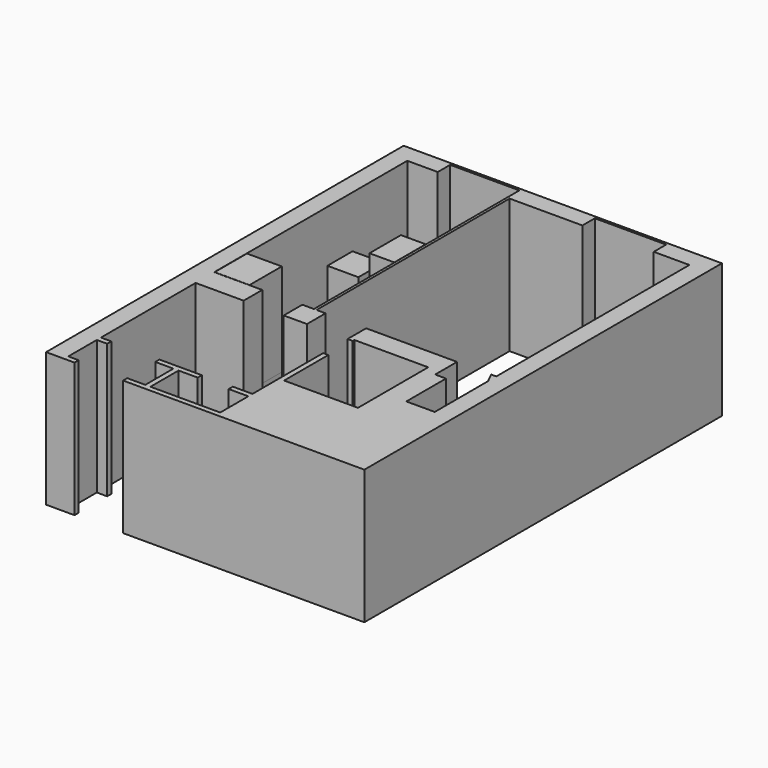
from build123d import *

# Parameters (mm, degrees)
F1_DEPTH = 800
F0_W     = 430
F0_H     = 1300
F0_W_2   = 220
F0_H_2   = 720
F0_W_3   = 480
F0_H_3   = 1200
F0_H_4   = 760
F0_W_4   = 675
F0_H_5   = 780
F0_W_5   = 600
F0_H_6   = 531.0021286011
F0_H_7   = 100
F0_H_8   = 1304.4725608826
F0_H_9   = 607.3201847076
F0_W_6   = 642.8868770599
F0_H_10  = 620.1963424683
F2_DEPTH = 1200
F3_DEPTH = 800
F4_DEPTH = 1800


with BuildPart() as f1:
    # F0 (on Top) → F1 (new body)
    with BuildSketch(Plane.XY):
        Polygon((0, -3630), (0, 5020), (-6160, 5020), (-6160, -3630), (-5810, -3630), (-5610, -3630), (-5610, -3530), (-5810, -3530), (-5810, -2840), (-5610, -2840), (-5610, -2740), (-5810, -2740), (-5810, -450), (-4880, -450), (-4880, 0), (-5810, 0), (-5810, 4670), (-5220, 4670), (-5220, 4970), (-3880, 4970), (-3880, 4670), (-3880, 0), (-4105, 0), (-4105, -450), (-3655, -450), (-3655, 0), (-3830, 0), (-3830, 4670), (-2420, 4670), (-2420, 4970), (-1040, 4970), (-1040, 4670), (-350, 4670), (-350, 0), (-450, 0), (-350, -200), (-350, -1490), (-900, -1490), (-900, -530), (-1110, -530), (-1110, 0), (-2870, 0), (-2870, -450), (-2770, -450), (-2770, -410), (-1340, -410), (-1340, -2110), (-2770, -2110), (-2770, -1040), (-2870, -1040), (-2870, -2750), (-3250, -2750), (-3250, -2850), (-2870, -2850), (-2870, -3530), (-4220, -3530), (-4220, -2850), (-3850, -2850), (-3850, -2750), (-4670, -2750), (-4670, -2850), (-4320, -2850), (-4320, -3530), (-4670, -3530), (-4670, -3630), (-4320, -3630), align=None)
    extrude(amount=F1_DEPTH)

    # F4 (add): a face of the model
    f4_faces = [f1.faces().sort_by_distance(p)[0] for p in [
        (-2581.1160504996, -299.791944949, 800),
    ]]
    extrude(f4_faces, amount=F4_DEPTH)


with BuildPart() as f1b:
    # F0 (on Top) → F1, piece 2 (new body)
    with BuildSketch(Plane.XY):
        with Locations((-3095, -1790)):
            Rectangle(F0_W, F0_H)
    extrude(amount=F1_DEPTH)

    # F2 (add): a face of the model
    f2_faces = [f1b.faces().sort_by_distance(p)[0] for p in [
        (-3095, -1790, 800),
    ]]
    extrude(f2_faces, amount=F2_DEPTH)


with BuildPart() as f1c:
    # F0 (on Top) → F1, piece 3 (new body)
    with BuildSketch(Plane.XY):
        with Locations((-3995, 365)):
            Rectangle(F0_W_2, F0_H_2)
    extrude(amount=F1_DEPTH)


with BuildPart() as f1d:
    # F0 (on Top) → F1, piece 4 (new body)
    with BuildSketch(Plane.XY):
        with Locations((-4125, 1345)):
            Rectangle(F0_W_3, F0_H_3)
    extrude(amount=F1_DEPTH)


with BuildPart() as f1e:
    # F0 (on Top) → F1, piece 5 (new body)
    with BuildSketch(Plane.XY):
        with Locations((-4125, 2330)):
            Rectangle(F0_W_3, F0_H_4)
    extrude(amount=F1_DEPTH)


with BuildPart() as f1f:
    # F0 (on Top) → F1, piece 6 (new body)
    with BuildSketch(Plane.XY):
        with Locations((-5467.5, 395)):
            Rectangle(F0_W_4, F0_H_5)
    extrude(amount=F1_DEPTH)


with BuildPart() as f1g:
    # F0 (on Top) → F1, piece 7 (new body)
    with BuildSketch(Plane.XY):
        with Locations((-5505, 1152.5010643005)):
            Rectangle(F0_W_5, F0_H_6)
    extrude(amount=F1_DEPTH)


with BuildPart() as f1h:
    # F0 (on Top) → F1, piece 8 (new body)
    with BuildSketch(Plane.XY):
        with Locations((-5505, 836)):
            Rectangle(F0_W_5, F0_H_7)
    extrude(amount=F1_DEPTH)


with BuildPart() as f1i:
    # F0 (on Top) → F1, piece 9 (new body)
    with BuildSketch(Plane.XY):
        with Locations((-5505, 2075.2384090424)):
            Rectangle(F0_W_5, F0_H_8)
    extrude(amount=F1_DEPTH)


with BuildPart() as f1j:
    # F0 (on Top) → F1, piece 10 (new body)
    with BuildSketch(Plane.XY):
        with Locations((-5505, 3036.1347818375)):
            Rectangle(F0_W_5, F0_H_9)
    extrude(amount=F1_DEPTH)

    # F3 (add): a face of the model
    f3_faces = [f1j.faces().sort_by_distance(p)[0] for p in [
        (-5505, 3036.1347818375, 800),
    ]]
    extrude(f3_faces, amount=F3_DEPTH)


with BuildPart() as f1k:
    # F0 (on Top) → F1, piece 11 (new body)
    with BuildSketch(Plane.XY):
        with Locations((-4288.8666391373, 3931.1900138855)):
            Rectangle(F0_W_6, F0_H_10)
    extrude(amount=F1_DEPTH)


with BuildPart() as f1l:
    # F0 (on Top) → F1, piece 12 (new body)
    with BuildSketch(Plane.XY):
        with BuildLine():
            ThreePointArc((-4416.8108707663, 3501.328542291), (-4430.368811286, 3497.3058256885), (-4426.3460946835, 3483.7478851687))
            ThreePointArc((-4426.3460946835, 3483.7478851687), (-4275.2294540405, 3445.4055272516), (-4124.1128133976, 3483.7478851687))
            ThreePointArc((-4124.1128133976, 3483.7478851687), (-4120.0900967951, 3497.3058256885), (-4133.6480373148, 3501.328542291))
            ThreePointArc((-4133.6480373148, 3501.328542291), (-4275.2294540405, 3465.4055272516), (-4416.8108707663, 3501.328542291))
        make_face()
    extrude(amount=F1_DEPTH)


with BuildPart() as f1m:
    # F0 (on Top) → F1, piece 13 (new body)
    with BuildSketch(Plane.XY):
        with BuildLine():
            ThreePointArc((-4416.8108707663, 4361.05148548), (-4275.2294540405, 4396.9745005194), (-4133.6480373148, 4361.05148548))
            ThreePointArc((-4133.6480373148, 4361.05148548), (-4120.0900967951, 4365.0742020825), (-4124.1128133976, 4378.6321426022))
            ThreePointArc((-4124.1128133976, 4378.6321426022), (-4275.2294540405, 4416.9745005194), (-4426.3460946835, 4378.6321426022))
            ThreePointArc((-4426.3460946835, 4378.6321426022), (-4430.368811286, 4365.0742020825), (-4416.8108707663, 4361.05148548))
        make_face()
    extrude(amount=F1_DEPTH)


with BuildPart() as f2:
    # F2#2 (new): a face of the model
    f2_2_faces = [f1c.part.faces().sort_by_distance(p)[0] for p in [
        (-3995, 365, 800),
    ]]
    extrude(f2_2_faces, amount=F2_DEPTH)


with BuildPart() as f4:
    # F4#2 (new): a face of the model
    f4_2_faces = [f1f.part.faces().sort_by_distance(p)[0] for p in [
        (-5467.5, 395, 800),
    ]]
    extrude(f4_2_faces, amount=F4_DEPTH)


with BuildPart() as f4b:
    # F4#3 (new): a face of the model
    f4_3_faces = [f1e.part.faces().sort_by_distance(p)[0] for p in [
        (-4125, 2330, 800),
    ]]
    extrude(f4_3_faces, amount=F4_DEPTH)


solid = Compound([f1.part, f1b.part, f1c.part, f1d.part, f1e.part, f1f.part, f1g.part, f1h.part, f1i.part, f1j.part, f1k.part, f1l.part, f1m.part, f2.part, f4.part, f4b.part])
